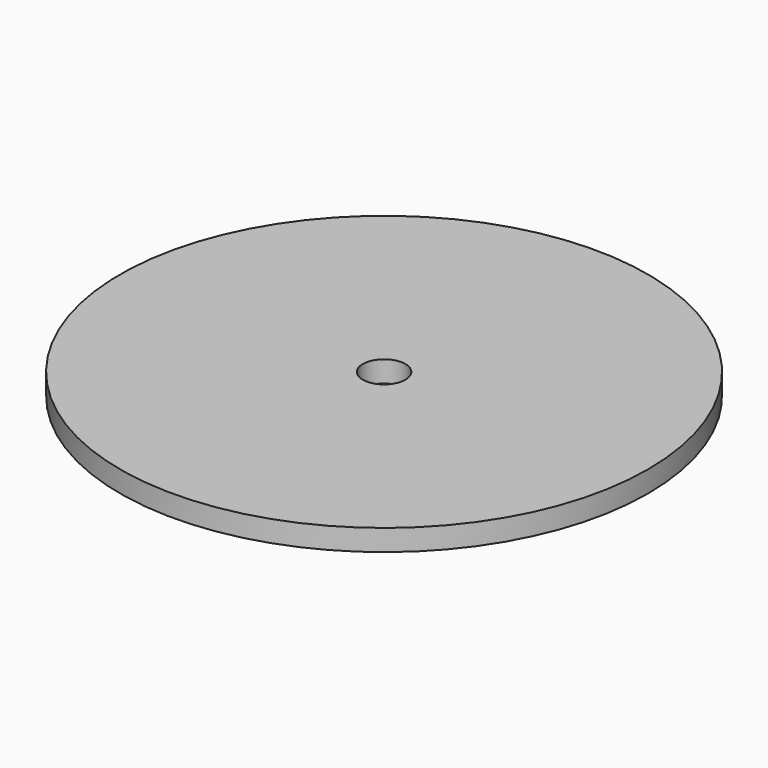
from build123d import *

# Parameters (mm, degrees)
F0_R     = 62
F3_DEPTH = 5
F1_R     = 5
F4_DEPTH = 25


# Not quite as in the source:
# - the program builds the solid bodies; features that only make, move or delete a surface that nothing else refers to are left out


with BuildPart() as f3:
    # F0 (on Top) → F3 (new body)
    with BuildSketch(Plane.XY):
        Circle(F0_R)
    extrude(amount=-F3_DEPTH)

    # F1 (on Top) → F4 (cut)
    with BuildSketch(Plane.XY):
        Circle(F1_R)
    extrude(amount=-F4_DEPTH, mode=Mode.SUBTRACT)


solid = f3.part
